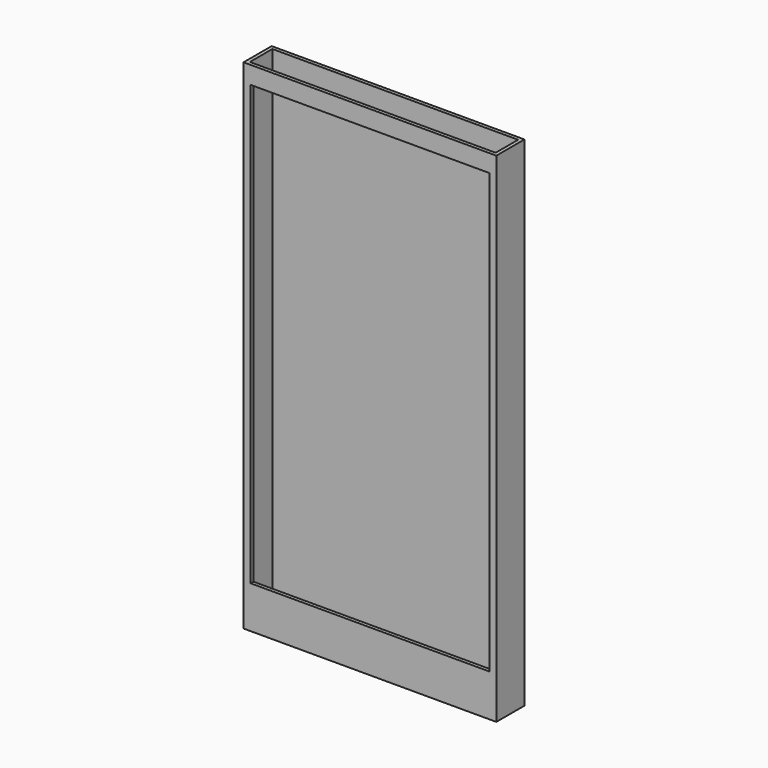
from build123d import *

# Parameters (mm, degrees)
F0_W     = 72
F0_H     = 142
F1_DEPTH = 10
F2_W     = 70
F2_H     = 8
F3_DEPTH = 140
F4_W     = 68
F4_H     = 125
F5_DEPTH = 4
F6_W     = 15
F6_H     = 3.25
F6_R     = 2.5
F7_DEPTH = 5
F9_DEPTH = 57


# Not quite as in the source:
# - ends of sketch curves that miss each other by under 0.0002 mm in the source are joined


with BuildPart() as f1:
    # F0 (on Front) → F1 (new body)
    with BuildSketch(Plane.XZ):
        with Locations((-12.5587194562, -2.6913457513)):
            Rectangle(F0_W, F0_H)
    extrude(amount=F1_DEPTH)

    # F2 (on face) → F3 (cut)
    with BuildSketch(Plane.XY.offset(68.3086542487)):
        with Locations((-12.5587194562, -5)):
            Rectangle(F2_W, F2_H)
    extrude(amount=-F3_DEPTH, mode=Mode.SUBTRACT)

    # F4 (on face) → F5 (cut)
    with BuildSketch(Plane.XZ.offset(10)):
        with Locations((-12.5587194562, 0.8086542487)):
            Rectangle(F4_W, F4_H)
    extrude(amount=-F5_DEPTH, mode=Mode.SUBTRACT)

    # F6 (on face) → F7 (cut)
    with BuildSketch(Plane(origin=(0, 0, -73.6913457513), x_dir=(1, 0, 0), z_dir=(0, 0, -1))):
        with Locations((-12.5587194562, 4.375)):
            Rectangle(F6_W, F6_H)
        with Locations((-32.8787194562, 4.5)):
            Circle(F6_R)
    extrude(amount=-F7_DEPTH, mode=Mode.SUBTRACT)


with BuildPart() as f9:
    # F8 (on Top) → F9 (new body, symmetric)
    with BuildSketch(Plane.XY):
        with BuildLine():
            ThreePointArc((7.7113736967, 14.9379451755), (-7.3445934288, 1.7428756888), (-23.4948524625, 13.5733929211))
            Line((-23.4948524625, 13.5733929211), (-26.0410183017, 13.4449196816))
            ThreePointArc((-26.0410183017, 13.4449196816), (-21.4884748179, 5.0199592107), (-13.3333762735, 1.1589e-06))
            Line((-13.3333762735, 1.1589e-06), (-13.2333813235, 1.1589e-06))
            Line((-13.2333813235, 1.1589e-06), (-3.3333762735, 0))
            ThreePointArc((-3.3333762735, 0), (5.0947085652, 4.9276153802), (9.8008521931, 13.4813408573))
            Line((9.8008521931, 13.4813408573), (7.7113736967, 14.9379451755))
        make_face()
    extrude(amount=F9_DEPTH, both=True)


with BuildPart() as f9_1:
    # F10: moved
    add(f9.part.moved(Location((-5.2, 0, 0))))


solid = Compound([f1.part, f9_1.part])
